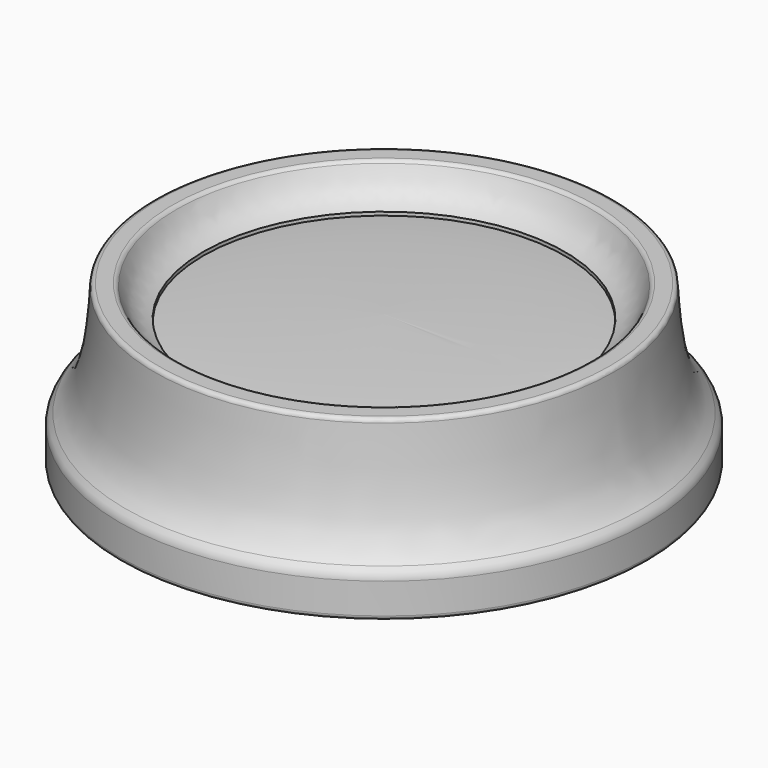
from build123d import *

# Parameters (mm, degrees)
F0_R     = 5.9
F0_R_2   = 5.1
F0_R_3   = 4.9
F1_DEPTH = 8
F3_R     = 13
F3_R_2   = 5.9
F4_DEPTH = 1.5
F5_W     = 13
F5_H     = 1.2751376927
F9_R     = 0.3
F10_R    = 3
F11_SIZE = 0.25


with BuildPart() as f1:
    # F0 (on Top) → F1 (new body)
    with BuildSketch(Plane.XY):
        Circle(F0_R)
        Circle(F0_R_2, mode=Mode.SUBTRACT)
        Circle(F0_R_2)
        Circle(F0_R_3, mode=Mode.SUBTRACT)
        Circle(F0_R_3)
        with BuildLine():
            ThreePointArc((-3.4278273002, -1.1), (-0.5566963801, 3.5566963801), (3.6, 0))
            ThreePointArc((3.6, 0), (3.5566963801, -0.5566963801), (3.4278273002, -1.1))
            ThreePointArc((3.4278273002, -1.1), (2.5187341799, -2.5721543755), (1.0278273002, -3.4501552198))
            ThreePointArc((1.0278273002, -3.4501552198), (0.519346324, -3.5623418415), (0, -3.6))
            ThreePointArc((0, -3.6), (-0.519346324, -3.5623418415), (-1.0278273002, -3.4501552198))
            ThreePointArc((-1.0278273002, -3.4501552198), (-2.5187341799, -2.5721543755), (-3.4278273002, -1.1))
        make_face(mode=Mode.SUBTRACT)
        with BuildLine():
            Line((-1.0278273002, -1.1), (-3.4278273002, -1.1))
            ThreePointArc((-3.4278273002, -1.1), (-2.5187341799, -2.5721543755), (-1.0278273002, -3.4501552198))
            Line((-1.0278273002, -3.4501552198), (-1.0278273002, -1.1))
        make_face()
        with BuildLine():
            ThreePointArc((1.0278273002, -3.4501552198), (2.5187341799, -2.5721543755), (3.4278273002, -1.1))
            Line((3.4278273002, -1.1), (1.0278273002, -1.1))
            Line((1.0278273002, -1.1), (1.0278273002, -3.4501552198))
        make_face()
    extrude(amount=F1_DEPTH)

    # F3 (on offset) → F4 (join)
    with BuildSketch(Plane.XY.offset(8)):
        Circle(F3_R)
        Circle(F3_R_2, mode=Mode.SUBTRACT)
        Circle(F3_R_2)
    extrude(amount=F4_DEPTH)

    # F5 (on Front) → F6 (revolve, cut)
    with BuildSketch(Plane.XZ):
        with Locations((6.5, 10.1375688463)):
            Rectangle(F5_W, F5_H)
        with BuildLine():
            Line((13, 9.5), (0, 9.5))
            add(Edge.make_bspline(
                [(0, 9.5), (4.7778501175, 9.4541264698), (10.4964841157, 9.2799523845), (13, 9)],
                knots=[0, 0, 0, 0, 13.0096118313, 13.0096118313, 13.0096118313, 13.0096118313], degree=3))
            Line((13, 9), (13, 9.5))
        make_face()
    revolve(axis=Axis((0, 0, 8), (0, 0, -1)), mode=Mode.SUBTRACT)

    # F7 (on Front) → F8 (revolve)
    with BuildSketch(Plane.XZ):
        with BuildLine():
            Line((18.6, 2.5), (19, 2.5))
            add(Edge.make_bspline(
                [(18.6, 3.25), (18.7663344502, 3.0912196208), (19, 2.8213595506), (19, 2.5)],
                knots=[0, 0, 0, 0, 0.85, 0.85, 0.85, 0.85], degree=3))
            Line((18.6, 3.25), (18.6, 2.5))
        make_face()
        with BuildLine():
            add(Edge.make_bspline(
                [(13, 8), (14.7166289389, 5.7283868082), (16.1443110555, 2.8730242047), (17, 0)],
                knots=[0, 0, 0, 0, 8.94427191, 8.94427191, 8.94427191, 8.94427191], degree=3))
            Line((17, 0), (19, 0))
            Line((19, 0), (19, 2.5))
            Line((19, 2.5), (18.6, 2.5))
            Line((18.6, 2.5), (18.6, 3.25))
            add(Edge.make_bspline(
                [(16.5, 11.5), (16.7500618845, 6.6030700691), (17.3276124358, 4.2607626356), (18.6, 3.25)],
                knots=[0, 0, 0, 0, 8.5130781742, 8.5130781742, 8.5130781742, 8.5130781742], degree=3))
            Line((16.5, 11.5), (15, 11.5))
            add(Edge.make_bspline(
                [(13, 9.25), (14.0098445117, 9.6409134567), (14.5036391914, 10.2233383805), (15, 11.5)],
                knots=[0, 0, 0, 0, 3.0103986447, 3.0103986447, 3.0103986447, 3.0103986447], degree=3))
            Line((13, 9.25), (13, 9))
            Line((13, 9), (13, 8))
        make_face()
    revolve(axis=Axis((0, 0, 8), (0, 0, -1)))

    # F9
    f9_edges = [f1.edges().sort_by_distance(p)[0] for p in [
        (-16.5, 0, 11.5),
        (-15, 0, 11.5),
        (-19, 0, 0),
        (-17, 0, 0),
    ]]
    fillet(f9_edges, radius=F9_R)

    # F10
    f10_edges = [f1.edges().sort_by_distance(p)[0] for p in [
        (-5.9, 0, 8),
        (-13, 0, 8),
    ]]
    fillet(f10_edges, radius=F10_R)

    # F11
    f11_edges = [f1.edges().sort_by_distance(p)[0] for p in [
        (-2.227827, -1.1, 0),
        (-1.027827, -2.275078, 0),
        (1.027827, -2.275078, 0),
        (2.227827, -1.1, 0),
        (0, -3.6, 0),
        (0, 3.6, 0),
    ]]
    chamfer(f11_edges, length=F11_SIZE)


solid = f1.part
